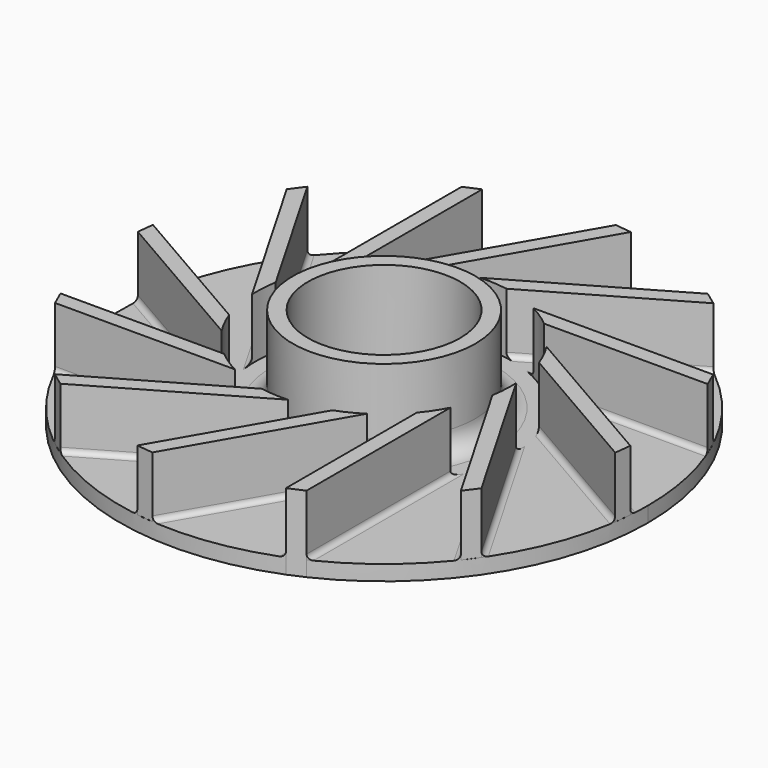
from build123d import *

# Parameters (mm, degrees)
F0_R          = 9
F0_R_2        = 7.5
F1_DEPTH      = 1.5
F2_DEPTH      = 7.5
F3_DEPTH      = 10
F4_COUNT      = 12
F6_T4_DEPTH   = 20.2062125085
F6_S5_R       = 26
F6_T6_DEPTH   = 12
F6_S7_R       = 12.5604672282
F6_T8_DEPTH   = 12
F6_T12_DEPTH  = 20.2062125085
F6_S13_R      = 26
F6_T14_DEPTH  = 12
F6_S15_R      = 12.5604672282
F6_T16_DEPTH  = 12
F6_T20_DEPTH  = 20.2062125085
F6_S21_R      = 26
F6_T22_DEPTH  = 12
F6_S23_R      = 12.5604672282
F6_T24_DEPTH  = 12
F6_T28_DEPTH  = 20.2062125085
F6_S29_R      = 26
F6_T30_DEPTH  = 12
F6_S31_R      = 12.5604672282
F6_T32_DEPTH  = 12
F6_T36_DEPTH  = 18.6035363085
F6_S37_R      = 12.5604672282
F6_T38_DEPTH  = 11
F6_S39_R      = 26
F6_T40_DEPTH  = 11
F6_T44_DEPTH  = 18.6035363085
F6_S45_R      = 12.5604672282
F6_T46_DEPTH  = 11
F6_S47_R      = 26
F6_T48_DEPTH  = 11
F6_T52_DEPTH  = 18.6035363085
F6_S53_R      = 12.5604672282
F6_T54_DEPTH  = 11
F6_S55_R      = 26
F6_T56_DEPTH  = 11
F6_T60_DEPTH  = 18.6035363085
F6_S61_R      = 12.5604672282
F6_T62_DEPTH  = 11
F6_S63_R      = 26
F6_T64_DEPTH  = 11
F6_T68_DEPTH  = 18.6035363085
F6_S69_R      = 12.5604672282
F6_T70_DEPTH  = 11
F6_S71_R      = 26
F6_T72_DEPTH  = 11
F6_T76_DEPTH  = 18.6035363085
F6_S77_R      = 12.5604672282
F6_T78_DEPTH  = 11
F6_S79_R      = 26
F6_T80_DEPTH  = 11
F6_T84_DEPTH  = 20.2062125085
F6_S85_R      = 26
F6_T86_DEPTH  = 12
F6_S87_R      = 12.5604672282
F6_T88_DEPTH  = 12
F6_T92_DEPTH  = 20.2062125085
F6_S93_R      = 26
F6_T94_DEPTH  = 12
F6_S95_R      = 12.5604672282
F6_T96_DEPTH  = 12
F6_T100_DEPTH = 20.2062125085
F6_S101_R     = 26
F6_T102_DEPTH = 12
F6_S103_R     = 12.5604672282
F6_T104_DEPTH = 12
F6_T108_DEPTH = 20.2062125085
F6_S109_R     = 26
F6_T110_DEPTH = 12
F6_S111_R     = 12.5604672282
F6_T112_DEPTH = 12
F6_T116_DEPTH = 20.2062125085
F6_S117_R     = 26
F6_T118_DEPTH = 12
F6_S119_R     = 12.5604672282
F6_T120_DEPTH = 12
F6_T124_DEPTH = 18.6035363085
F6_S125_R     = 12.5604672282
F6_T126_DEPTH = 11
F6_S127_R     = 26
F6_T128_DEPTH = 11
F6_T132_DEPTH = 18.6035363085
F6_S133_R     = 12.5604672282
F6_T134_DEPTH = 11
F6_S135_R     = 26
F6_T136_DEPTH = 11
F6_T140_DEPTH = 18.6035363085
F6_S141_R     = 12.5604672282
F6_T142_DEPTH = 11
F6_S143_R     = 26
F6_T144_DEPTH = 11
F6_T148_DEPTH = 18.6035363085
F6_S149_R     = 12.5604672282
F6_T150_DEPTH = 11
F6_S151_R     = 26
F6_T152_DEPTH = 11
F6_T156_DEPTH = 18.6035363085
F6_S157_R     = 12.5604672282
F6_T158_DEPTH = 11
F6_S159_R     = 26
F6_T160_DEPTH = 11
F6_T164_DEPTH = 18.6035363085
F6_S165_R     = 12.5604672282
F6_T166_DEPTH = 11
F6_S167_R     = 26
F6_T168_DEPTH = 11
F6_T172_DEPTH = 20.2062125085
F6_S173_R     = 26
F6_T174_DEPTH = 12
F6_S175_R     = 12.5604672282
F6_T176_DEPTH = 12
F6_T180_DEPTH = 20.2062125085
F6_S181_R     = 12.5604672282
F6_T182_DEPTH = 12
F6_S183_R     = 26
F6_T184_DEPTH = 12
F6_T188_DEPTH = 20.2062125085
F6_S189_R     = 26
F6_T190_DEPTH = 12
F6_S191_R     = 12.5604672282
F6_T192_DEPTH = 12
F7_R          = 2


# Not quite as in the source:
# - a fillet or chamfer that OpenCascade refuses, or shapes differently, is made with other operations: its cross-section is extruded or revolved along the edge and cut away or added


with BuildPart() as f1:
    # F0 (on Top) → F1 (new body)
    with BuildSketch(Plane.XY):
        with BuildLine():
            ThreePointArc((11.1509456635, -23.4873670472), (21.9764031094, -13.8938010053), (26, 0))
            ThreePointArc((26, 0), (-21.5281744146, 14.5786729977), (9.6509456635, -24.1424780791))
            Line((9.6509456635, -24.1424780791), (9.6509456635, -23.4873670472))
            Line((9.6509456635, -23.4873670472), (9.6509456635, -8.0389417706))
            ThreePointArc((9.6509456635, -8.0389417706), (10.462029989, -6.9506305829), (11.1509456635, -5.7811545388))
            Line((11.1509456635, -5.7811545388), (11.1509456635, -23.4873670472))
        make_face()
        Circle(F0_R, mode=Mode.SUBTRACT)
        Circle(F0_R)
        Circle(F0_R_2, mode=Mode.SUBTRACT)
    extrude(amount=F1_DEPTH)

    # F0 (on Top) → F3 (join)
    with BuildSketch(Plane.XY):
        Circle(F0_R)
        Circle(F0_R_2, mode=Mode.SUBTRACT)
    extrude(amount=F3_DEPTH)


with BuildPart() as f2:
    # F0 (on Top) → F2 (new body)
    with BuildSketch(Plane.XY):
        with BuildLine():
            Line((9.6509456635, -23.4873670472), (9.6509456635, -24.1424780791))
            Line((9.6509456635, -24.1424780791), (11.1509456635, -23.4873670472))
            Line((11.1509456635, -23.4873670472), (11.1509456635, -5.7811545388))
            ThreePointArc((11.1509456635, -5.7811545388), (10.462029989, -6.9506305829), (9.6509456635, -8.0389417706))
            Line((9.6509456635, -8.0389417706), (9.6509456635, -23.4873670472))
        make_face()
    extrude(amount=F2_DEPTH)


with BuildPart() as f4_1:
    # F4: instance of F2
    add(f2.part.rotate(Axis((0, 0, 0), (0, 0, 1)), 1 * 360 / F4_COUNT))


with BuildPart() as f4_2:
    # F4: instance of F2
    add(f2.part.rotate(Axis((0, 0, 0), (0, 0, 1)), 2 * 360 / F4_COUNT))


with BuildPart() as f4_3:
    # F4: instance of F2
    add(f2.part.rotate(Axis((0, 0, 0), (0, 0, 1)), 3 * 360 / F4_COUNT))


with BuildPart() as f4_4:
    # F4: instance of F2
    add(f2.part.rotate(Axis((0, 0, 0), (0, 0, 1)), 4 * 360 / F4_COUNT))


with BuildPart() as f4_5:
    # F4: instance of F2
    add(f2.part.rotate(Axis((0, 0, 0), (0, 0, 1)), 5 * 360 / F4_COUNT))


with BuildPart() as f4_6:
    # F4: instance of F2
    add(f2.part.rotate(Axis((0, 0, 0), (0, 0, 1)), 6 * 360 / F4_COUNT))


with BuildPart() as f4_7:
    # F4: instance of F2
    add(f2.part.rotate(Axis((0, 0, 0), (0, 0, 1)), 7 * 360 / F4_COUNT))


with BuildPart() as f4_8:
    # F4: instance of F2
    add(f2.part.rotate(Axis((0, 0, 0), (0, 0, 1)), 8 * 360 / F4_COUNT))


with BuildPart() as f4_9:
    # F4: instance of F2
    add(f2.part.rotate(Axis((0, 0, 0), (0, 0, 1)), 9 * 360 / F4_COUNT))


with BuildPart() as f4_10:
    # F4: instance of F2
    add(f2.part.rotate(Axis((0, 0, 0), (0, 0, 1)), 10 * 360 / F4_COUNT))


with BuildPart() as f4_11:
    # F4: instance of F2
    add(f2.part.rotate(Axis((0, 0, 0), (0, 0, 1)), 11 * 360 / F4_COUNT))


with BuildPart() as f1_1:
    add(f1.part)

    # F5: union F4_1, F4_2, F2, F4_3, F4_4, F4_5, F4_6, F4_7, F4_8, F4_9, F4_10, F4_11
    add(f4_1.part)
    add(f4_2.part)
    add(f2.part)
    add(f4_3.part)
    add(f4_4.part)
    add(f4_5.part)
    add(f4_6.part)
    add(f4_7.part)
    add(f4_8.part)
    add(f4_9.part)
    add(f4_10.part)
    add(f4_11.part)

    # F6: fillet of radius 0.5 on 24 edges, made by hand


with BuildPart() as f6_tool2:
    # F6_s3 → F6_t4 (new body)
    with BuildSketch(Plane(origin=(-2.2655772694, 3.924094939, 0), x_dir=(0, 0, 1), z_dir=(-0.5, 0.8660254038, 0))):
        with BuildLine():
            ThreePointArc((1.5, -11.6509456635), (1.6464466094, -11.2973922729), (2, -11.1509456635))
            Line((2, -11.1509456635), (1.5, -11.1509456635))
            Line((1.5, -11.1509456635), (1.5, -11.6509456635))
        make_face()
    extrude(amount=F6_T4_DEPTH)

    # F6_s5 → F6_t6 (intersect, symmetric)
    with BuildSketch(Plane.XY.offset(1.8)):
        Circle(F6_S5_R)
    extrude(amount=F6_T6_DEPTH, both=True, mode=Mode.INTERSECT)

    # F6_s7 → F6_t8 (cut, symmetric)
    with BuildSketch(Plane.XY.offset(1.8)):
        Circle(F6_S7_R)
    extrude(amount=F6_T8_DEPTH, both=True, mode=Mode.SUBTRACT)


with BuildPart() as f1_2:
    add(f1_1.part)

    # F6_t1: union F6_tool2
    add(f6_tool2.part)


with BuildPart() as f6_tool10:
    # F6_s11 → F6_t12 (new body)
    with BuildSketch(Plane(origin=(-3.924094939, 2.2655772694, 0), x_dir=(0, 0, 1), z_dir=(-0.8660254038, 0.5, 0))):
        with BuildLine():
            ThreePointArc((1.5, -11.6509456635), (1.6464466094, -11.2973922729), (2, -11.1509456635))
            Line((2, -11.1509456635), (1.5, -11.1509456635))
            Line((1.5, -11.1509456635), (1.5, -11.6509456635))
        make_face()
    extrude(amount=F6_T12_DEPTH)

    # F6_s13 → F6_t14 (intersect, symmetric)
    with BuildSketch(Plane.XY.offset(1.8)):
        Circle(F6_S13_R)
    extrude(amount=F6_T14_DEPTH, both=True, mode=Mode.INTERSECT)

    # F6_s15 → F6_t16 (cut, symmetric)
    with BuildSketch(Plane.XY.offset(1.8)):
        Circle(F6_S15_R)
    extrude(amount=F6_T16_DEPTH, both=True, mode=Mode.SUBTRACT)


with BuildPart() as f1_3:
    add(f1_2.part)

    # F6_t9: union F6_tool10
    add(f6_tool10.part)


with BuildPart() as f6_tool18:
    # F6_s19 → F6_t20 (new body)
    with BuildSketch(Plane.YZ.offset(-4.5311545388)):
        with BuildLine():
            ThreePointArc((-11.6509456635, 1.5), (-11.2973922729, 1.6464466094), (-11.1509456635, 2))
            Line((-11.1509456635, 2), (-11.1509456635, 1.5))
            Line((-11.1509456635, 1.5), (-11.6509456635, 1.5))
        make_face()
    extrude(amount=-F6_T20_DEPTH)

    # F6_s21 → F6_t22 (intersect, symmetric)
    with BuildSketch(Plane.XY.offset(1.8)):
        Circle(F6_S21_R)
    extrude(amount=F6_T22_DEPTH, both=True, mode=Mode.INTERSECT)

    # F6_s23 → F6_t24 (cut, symmetric)
    with BuildSketch(Plane.XY.offset(1.8)):
        Circle(F6_S23_R)
    extrude(amount=F6_T24_DEPTH, both=True, mode=Mode.SUBTRACT)


with BuildPart() as f1_4:
    add(f1_3.part)

    # F6_t17: union F6_tool18
    add(f6_tool18.part)


with BuildPart() as f6_tool26:
    # F6_s27 → F6_t28 (new body)
    with BuildSketch(Plane(origin=(-3.924094939, -2.2655772694, 0), x_dir=(0, 0, 1), z_dir=(-0.8660254038, -0.5, 0))):
        with BuildLine():
            ThreePointArc((1.5, -11.6509456635), (1.6464466094, -11.2973922729), (2, -11.1509456635))
            Line((2, -11.1509456635), (1.5, -11.1509456635))
            Line((1.5, -11.1509456635), (1.5, -11.6509456635))
        make_face()
    extrude(amount=F6_T28_DEPTH)

    # F6_s29 → F6_t30 (intersect, symmetric)
    with BuildSketch(Plane.XY.offset(1.8)):
        Circle(F6_S29_R)
    extrude(amount=F6_T30_DEPTH, both=True, mode=Mode.INTERSECT)

    # F6_s31 → F6_t32 (cut, symmetric)
    with BuildSketch(Plane.XY.offset(1.8)):
        Circle(F6_S31_R)
    extrude(amount=F6_T32_DEPTH, both=True, mode=Mode.SUBTRACT)


with BuildPart() as f1_5:
    add(f1_4.part)

    # F6_t25: union F6_tool26
    add(f6_tool26.part)


with BuildPart() as f6_tool34:
    # F6_s35 → F6_t36 (new body)
    with BuildSketch(Plane(origin=(-21.9905310816, 12.6962390396, 0), x_dir=(0, 0, 1), z_dir=(0.8660254038, -0.5, 0))):
        with BuildLine():
            ThreePointArc((1.5, 9.1509456635), (1.6464466094, 9.504499054), (2, 9.6509456635))
            Line((2, 9.6509456635), (1.5, 9.6509456635))
            Line((1.5, 9.6509456635), (1.5, 9.1509456635))
        make_face()
    extrude(amount=F6_T36_DEPTH)

    # F6_s37 → F6_t38 (cut, symmetric)
    with BuildSketch(Plane.XY.offset(1.8)):
        Circle(F6_S37_R)
    extrude(amount=F6_T38_DEPTH, both=True, mode=Mode.SUBTRACT)

    # F6_s39 → F6_t40 (intersect, symmetric)
    with BuildSketch(Plane.XY.offset(1.8)):
        Circle(F6_S39_R)
    extrude(amount=F6_T40_DEPTH, both=True, mode=Mode.INTERSECT)


with BuildPart() as f1_6:
    add(f1_5.part)

    # F6_t33: union F6_tool34
    add(f6_tool34.part)


with BuildPart() as f6_tool42:
    # F6_s43 → F6_t44 (new body)
    with BuildSketch(Plane.YZ.offset(-25.3924780791)):
        with BuildLine():
            ThreePointArc((-9.1509456635, 1.5), (-9.504499054, 1.6464466094), (-9.6509456635, 2))
            Line((-9.6509456635, 2), (-9.6509456635, 1.5))
            Line((-9.6509456635, 1.5), (-9.1509456635, 1.5))
        make_face()
    extrude(amount=F6_T44_DEPTH)

    # F6_s45 → F6_t46 (cut, symmetric)
    with BuildSketch(Plane.XY.offset(1.8)):
        Circle(F6_S45_R)
    extrude(amount=F6_T46_DEPTH, both=True, mode=Mode.SUBTRACT)

    # F6_s47 → F6_t48 (intersect, symmetric)
    with BuildSketch(Plane.XY.offset(1.8)):
        Circle(F6_S47_R)
    extrude(amount=F6_T48_DEPTH, both=True, mode=Mode.INTERSECT)


with BuildPart() as f1_7:
    add(f1_6.part)

    # F6_t41: union F6_tool42
    add(f6_tool42.part)


with BuildPart() as f6_tool50:
    # F6_s51 → F6_t52 (new body)
    with BuildSketch(Plane(origin=(-21.9905310816, -12.6962390396, 0), x_dir=(0, 0, 1), z_dir=(0.8660254038, 0.5, 0))):
        with BuildLine():
            ThreePointArc((1.5, 9.1509456635), (1.6464466094, 9.504499054), (2, 9.6509456635))
            Line((2, 9.6509456635), (1.5, 9.6509456635))
            Line((1.5, 9.6509456635), (1.5, 9.1509456635))
        make_face()
    extrude(amount=F6_T52_DEPTH)

    # F6_s53 → F6_t54 (cut, symmetric)
    with BuildSketch(Plane.XY.offset(1.8)):
        Circle(F6_S53_R)
    extrude(amount=F6_T54_DEPTH, both=True, mode=Mode.SUBTRACT)

    # F6_s55 → F6_t56 (intersect, symmetric)
    with BuildSketch(Plane.XY.offset(1.8)):
        Circle(F6_S55_R)
    extrude(amount=F6_T56_DEPTH, both=True, mode=Mode.INTERSECT)


with BuildPart() as f1_8:
    add(f1_7.part)

    # F6_t49: union F6_tool50
    add(f6_tool50.part)


with BuildPart() as f6_tool58:
    # F6_s59 → F6_t60 (new body)
    with BuildSketch(Plane(origin=(-12.6962390396, -21.9905310816, 0), x_dir=(0, 0, 1), z_dir=(0.5, 0.8660254038, 0))):
        with BuildLine():
            ThreePointArc((1.5, 9.1509456635), (1.6464466094, 9.504499054), (2, 9.6509456635))
            Line((2, 9.6509456635), (1.5, 9.6509456635))
            Line((1.5, 9.6509456635), (1.5, 9.1509456635))
        make_face()
    extrude(amount=F6_T60_DEPTH)

    # F6_s61 → F6_t62 (cut, symmetric)
    with BuildSketch(Plane.XY.offset(1.8)):
        Circle(F6_S61_R)
    extrude(amount=F6_T62_DEPTH, both=True, mode=Mode.SUBTRACT)

    # F6_s63 → F6_t64 (intersect, symmetric)
    with BuildSketch(Plane.XY.offset(1.8)):
        Circle(F6_S63_R)
    extrude(amount=F6_T64_DEPTH, both=True, mode=Mode.INTERSECT)


with BuildPart() as f1_9:
    add(f1_8.part)

    # F6_t57: union F6_tool58
    add(f6_tool58.part)


with BuildPart() as f6_tool66:
    # F6_s67 → F6_t68 (new body)
    with BuildSketch(Plane.XZ.offset(25.3924780791)):
        with BuildLine():
            ThreePointArc((9.1509456635, 1.5), (9.504499054, 1.6464466094), (9.6509456635, 2))
            Line((9.6509456635, 2), (9.6509456635, 1.5))
            Line((9.6509456635, 1.5), (9.1509456635, 1.5))
        make_face()
    extrude(amount=-F6_T68_DEPTH)

    # F6_s69 → F6_t70 (cut, symmetric)
    with BuildSketch(Plane.XY.offset(1.8)):
        Circle(F6_S69_R)
    extrude(amount=F6_T70_DEPTH, both=True, mode=Mode.SUBTRACT)

    # F6_s71 → F6_t72 (intersect, symmetric)
    with BuildSketch(Plane.XY.offset(1.8)):
        Circle(F6_S71_R)
    extrude(amount=F6_T72_DEPTH, both=True, mode=Mode.INTERSECT)


with BuildPart() as f1_10:
    add(f1_9.part)

    # F6_t65: union F6_tool66
    add(f6_tool66.part)


with BuildPart() as f6_tool74:
    # F6_s75 → F6_t76 (new body)
    with BuildSketch(Plane(origin=(12.6962390396, -21.9905310816, 0), x_dir=(0, 0, 1), z_dir=(-0.5, 0.8660254038, 0))):
        with BuildLine():
            ThreePointArc((1.5, 9.1509456635), (1.6464466094, 9.504499054), (2, 9.6509456635))
            Line((2, 9.6509456635), (1.5, 9.6509456635))
            Line((1.5, 9.6509456635), (1.5, 9.1509456635))
        make_face()
    extrude(amount=F6_T76_DEPTH)

    # F6_s77 → F6_t78 (cut, symmetric)
    with BuildSketch(Plane.XY.offset(1.8)):
        Circle(F6_S77_R)
    extrude(amount=F6_T78_DEPTH, both=True, mode=Mode.SUBTRACT)

    # F6_s79 → F6_t80 (intersect, symmetric)
    with BuildSketch(Plane.XY.offset(1.8)):
        Circle(F6_S79_R)
    extrude(amount=F6_T80_DEPTH, both=True, mode=Mode.INTERSECT)


with BuildPart() as f1_11:
    add(f1_10.part)

    # F6_t73: union F6_tool74
    add(f6_tool74.part)


with BuildPart() as f6_tool82:
    # F6_s83 → F6_t84 (new body)
    with BuildSketch(Plane(origin=(3.924094939, -2.2655772694, 0), x_dir=(0, 0, 1), z_dir=(0.8660254038, -0.5, 0))):
        with BuildLine():
            ThreePointArc((1.5, -11.6509456635), (1.6464466094, -11.2973922729), (2, -11.1509456635))
            Line((2, -11.1509456635), (1.5, -11.1509456635))
            Line((1.5, -11.1509456635), (1.5, -11.6509456635))
        make_face()
    extrude(amount=F6_T84_DEPTH)

    # F6_s85 → F6_t86 (intersect, symmetric)
    with BuildSketch(Plane.XY.offset(1.8)):
        Circle(F6_S85_R)
    extrude(amount=F6_T86_DEPTH, both=True, mode=Mode.INTERSECT)

    # F6_s87 → F6_t88 (cut, symmetric)
    with BuildSketch(Plane.XY.offset(1.8)):
        Circle(F6_S87_R)
    extrude(amount=F6_T88_DEPTH, both=True, mode=Mode.SUBTRACT)


with BuildPart() as f1_12:
    add(f1_11.part)

    # F6_t81: union F6_tool82
    add(f6_tool82.part)


with BuildPart() as f6_tool90:
    # F6_s91 → F6_t92 (new body)
    with BuildSketch(Plane.YZ.offset(4.5311545388)):
        with BuildLine():
            ThreePointArc((11.6509456635, 1.5), (11.2973922729, 1.6464466094), (11.1509456635, 2))
            Line((11.1509456635, 2), (11.1509456635, 1.5))
            Line((11.1509456635, 1.5), (11.6509456635, 1.5))
        make_face()
    extrude(amount=F6_T92_DEPTH)

    # F6_s93 → F6_t94 (intersect, symmetric)
    with BuildSketch(Plane.XY.offset(1.8)):
        Circle(F6_S93_R)
    extrude(amount=F6_T94_DEPTH, both=True, mode=Mode.INTERSECT)

    # F6_s95 → F6_t96 (cut, symmetric)
    with BuildSketch(Plane.XY.offset(1.8)):
        Circle(F6_S95_R)
    extrude(amount=F6_T96_DEPTH, both=True, mode=Mode.SUBTRACT)


with BuildPart() as f1_13:
    add(f1_12.part)

    # F6_t89: union F6_tool90
    add(f6_tool90.part)


with BuildPart() as f6_tool98:
    # F6_s99 → F6_t100 (new body)
    with BuildSketch(Plane(origin=(3.924094939, 2.2655772694, 0), x_dir=(0, 0, 1), z_dir=(0.8660254038, 0.5, 0))):
        with BuildLine():
            ThreePointArc((1.5, -11.6509456635), (1.6464466094, -11.2973922729), (2, -11.1509456635))
            Line((2, -11.1509456635), (1.5, -11.1509456635))
            Line((1.5, -11.1509456635), (1.5, -11.6509456635))
        make_face()
    extrude(amount=F6_T100_DEPTH)

    # F6_s101 → F6_t102 (intersect, symmetric)
    with BuildSketch(Plane.XY.offset(1.8)):
        Circle(F6_S101_R)
    extrude(amount=F6_T102_DEPTH, both=True, mode=Mode.INTERSECT)

    # F6_s103 → F6_t104 (cut, symmetric)
    with BuildSketch(Plane.XY.offset(1.8)):
        Circle(F6_S103_R)
    extrude(amount=F6_T104_DEPTH, both=True, mode=Mode.SUBTRACT)


with BuildPart() as f1_14:
    add(f1_13.part)

    # F6_t97: union F6_tool98
    add(f6_tool98.part)


with BuildPart() as f6_tool106:
    # F6_s107 → F6_t108 (new body)
    with BuildSketch(Plane(origin=(2.2655772694, 3.924094939, 0), x_dir=(0, 0, 1), z_dir=(0.5, 0.8660254038, 0))):
        with BuildLine():
            ThreePointArc((1.5, -11.6509456635), (1.6464466094, -11.2973922729), (2, -11.1509456635))
            Line((2, -11.1509456635), (1.5, -11.1509456635))
            Line((1.5, -11.1509456635), (1.5, -11.6509456635))
        make_face()
    extrude(amount=F6_T108_DEPTH)

    # F6_s109 → F6_t110 (intersect, symmetric)
    with BuildSketch(Plane.XY.offset(1.8)):
        Circle(F6_S109_R)
    extrude(amount=F6_T110_DEPTH, both=True, mode=Mode.INTERSECT)

    # F6_s111 → F6_t112 (cut, symmetric)
    with BuildSketch(Plane.XY.offset(1.8)):
        Circle(F6_S111_R)
    extrude(amount=F6_T112_DEPTH, both=True, mode=Mode.SUBTRACT)


with BuildPart() as f1_15:
    add(f1_14.part)

    # F6_t105: union F6_tool106
    add(f6_tool106.part)


with BuildPart() as f6_tool114:
    # F6_s115 → F6_t116 (new body)
    with BuildSketch(Plane.XZ.offset(-4.5311545388)):
        with BuildLine():
            ThreePointArc((-11.6509456635, 1.5), (-11.2973922729, 1.6464466094), (-11.1509456635, 2))
            Line((-11.1509456635, 2), (-11.1509456635, 1.5))
            Line((-11.1509456635, 1.5), (-11.6509456635, 1.5))
        make_face()
    extrude(amount=-F6_T116_DEPTH)

    # F6_s117 → F6_t118 (intersect, symmetric)
    with BuildSketch(Plane.XY.offset(1.8)):
        Circle(F6_S117_R)
    extrude(amount=F6_T118_DEPTH, both=True, mode=Mode.INTERSECT)

    # F6_s119 → F6_t120 (cut, symmetric)
    with BuildSketch(Plane.XY.offset(1.8)):
        Circle(F6_S119_R)
    extrude(amount=F6_T120_DEPTH, both=True, mode=Mode.SUBTRACT)


with BuildPart() as f1_16:
    add(f1_15.part)

    # F6_t113: union F6_tool114
    add(f6_tool114.part)


with BuildPart() as f6_tool122:
    # F6_s123 → F6_t124 (new body)
    with BuildSketch(Plane.XZ.offset(-25.3924780791)):
        with BuildLine():
            ThreePointArc((-9.1509456635, 1.5), (-9.504499054, 1.6464466094), (-9.6509456635, 2))
            Line((-9.6509456635, 2), (-9.6509456635, 1.5))
            Line((-9.6509456635, 1.5), (-9.1509456635, 1.5))
        make_face()
    extrude(amount=F6_T124_DEPTH)

    # F6_s125 → F6_t126 (cut, symmetric)
    with BuildSketch(Plane.XY.offset(1.8)):
        Circle(F6_S125_R)
    extrude(amount=F6_T126_DEPTH, both=True, mode=Mode.SUBTRACT)

    # F6_s127 → F6_t128 (intersect, symmetric)
    with BuildSketch(Plane.XY.offset(1.8)):
        Circle(F6_S127_R)
    extrude(amount=F6_T128_DEPTH, both=True, mode=Mode.INTERSECT)


with BuildPart() as f1_17:
    add(f1_16.part)

    # F6_t121: union F6_tool122
    add(f6_tool122.part)


with BuildPart() as f6_tool130:
    # F6_s131 → F6_t132 (new body)
    with BuildSketch(Plane(origin=(-12.6962390396, 21.9905310816, 0), x_dir=(0, 0, 1), z_dir=(0.5, -0.8660254038, 0))):
        with BuildLine():
            ThreePointArc((1.5, 9.1509456635), (1.6464466094, 9.504499054), (2, 9.6509456635))
            Line((2, 9.6509456635), (1.5, 9.6509456635))
            Line((1.5, 9.6509456635), (1.5, 9.1509456635))
        make_face()
    extrude(amount=F6_T132_DEPTH)

    # F6_s133 → F6_t134 (cut, symmetric)
    with BuildSketch(Plane.XY.offset(1.8)):
        Circle(F6_S133_R)
    extrude(amount=F6_T134_DEPTH, both=True, mode=Mode.SUBTRACT)

    # F6_s135 → F6_t136 (intersect, symmetric)
    with BuildSketch(Plane.XY.offset(1.8)):
        Circle(F6_S135_R)
    extrude(amount=F6_T136_DEPTH, both=True, mode=Mode.INTERSECT)


with BuildPart() as f1_18:
    add(f1_17.part)

    # F6_t129: union F6_tool130
    add(f6_tool130.part)


with BuildPart() as f6_tool138:
    # F6_s139 → F6_t140 (new body)
    with BuildSketch(Plane(origin=(12.6962390396, 21.9905310816, 0), x_dir=(0, 0, 1), z_dir=(-0.5, -0.8660254038, 0))):
        with BuildLine():
            ThreePointArc((1.5, 9.1509456635), (1.6464466094, 9.504499054), (2, 9.6509456635))
            Line((2, 9.6509456635), (1.5, 9.6509456635))
            Line((1.5, 9.6509456635), (1.5, 9.1509456635))
        make_face()
    extrude(amount=F6_T140_DEPTH)

    # F6_s141 → F6_t142 (cut, symmetric)
    with BuildSketch(Plane.XY.offset(1.8)):
        Circle(F6_S141_R)
    extrude(amount=F6_T142_DEPTH, both=True, mode=Mode.SUBTRACT)

    # F6_s143 → F6_t144 (intersect, symmetric)
    with BuildSketch(Plane.XY.offset(1.8)):
        Circle(F6_S143_R)
    extrude(amount=F6_T144_DEPTH, both=True, mode=Mode.INTERSECT)


with BuildPart() as f1_19:
    add(f1_18.part)

    # F6_t137: union F6_tool138
    add(f6_tool138.part)


with BuildPart() as f6_tool146:
    # F6_s147 → F6_t148 (new body)
    with BuildSketch(Plane(origin=(21.9905310816, 12.6962390396, 0), x_dir=(0, 0, 1), z_dir=(-0.8660254038, -0.5, 0))):
        with BuildLine():
            ThreePointArc((1.5, 9.1509456635), (1.6464466094, 9.504499054), (2, 9.6509456635))
            Line((2, 9.6509456635), (1.5, 9.6509456635))
            Line((1.5, 9.6509456635), (1.5, 9.1509456635))
        make_face()
    extrude(amount=F6_T148_DEPTH)

    # F6_s149 → F6_t150 (cut, symmetric)
    with BuildSketch(Plane.XY.offset(1.8)):
        Circle(F6_S149_R)
    extrude(amount=F6_T150_DEPTH, both=True, mode=Mode.SUBTRACT)

    # F6_s151 → F6_t152 (intersect, symmetric)
    with BuildSketch(Plane.XY.offset(1.8)):
        Circle(F6_S151_R)
    extrude(amount=F6_T152_DEPTH, both=True, mode=Mode.INTERSECT)


with BuildPart() as f1_20:
    add(f1_19.part)

    # F6_t145: union F6_tool146
    add(f6_tool146.part)


with BuildPart() as f6_tool154:
    # F6_s155 → F6_t156 (new body)
    with BuildSketch(Plane.YZ.offset(25.3924780791)):
        with BuildLine():
            ThreePointArc((9.1509456635, 1.5), (9.504499054, 1.6464466094), (9.6509456635, 2))
            Line((9.6509456635, 2), (9.6509456635, 1.5))
            Line((9.6509456635, 1.5), (9.1509456635, 1.5))
        make_face()
    extrude(amount=-F6_T156_DEPTH)

    # F6_s157 → F6_t158 (cut, symmetric)
    with BuildSketch(Plane.XY.offset(1.8)):
        Circle(F6_S157_R)
    extrude(amount=F6_T158_DEPTH, both=True, mode=Mode.SUBTRACT)

    # F6_s159 → F6_t160 (intersect, symmetric)
    with BuildSketch(Plane.XY.offset(1.8)):
        Circle(F6_S159_R)
    extrude(amount=F6_T160_DEPTH, both=True, mode=Mode.INTERSECT)


with BuildPart() as f1_21:
    add(f1_20.part)

    # F6_t153: union F6_tool154
    add(f6_tool154.part)


with BuildPart() as f6_tool162:
    # F6_s163 → F6_t164 (new body)
    with BuildSketch(Plane(origin=(21.9905310816, -12.6962390396, 0), x_dir=(0, 0, 1), z_dir=(-0.8660254038, 0.5, 0))):
        with BuildLine():
            ThreePointArc((1.5, 9.1509456635), (1.6464466094, 9.504499054), (2, 9.6509456635))
            Line((2, 9.6509456635), (1.5, 9.6509456635))
            Line((1.5, 9.6509456635), (1.5, 9.1509456635))
        make_face()
    extrude(amount=F6_T164_DEPTH)

    # F6_s165 → F6_t166 (cut, symmetric)
    with BuildSketch(Plane.XY.offset(1.8)):
        Circle(F6_S165_R)
    extrude(amount=F6_T166_DEPTH, both=True, mode=Mode.SUBTRACT)

    # F6_s167 → F6_t168 (intersect, symmetric)
    with BuildSketch(Plane.XY.offset(1.8)):
        Circle(F6_S167_R)
    extrude(amount=F6_T168_DEPTH, both=True, mode=Mode.INTERSECT)


with BuildPart() as f1_22:
    add(f1_21.part)

    # F6_t161: union F6_tool162
    add(f6_tool162.part)


with BuildPart() as f6_tool170:
    # F6_s171 → F6_t172 (new body)
    with BuildSketch(Plane(origin=(2.2655772694, -3.924094939, 0), x_dir=(0, 0, 1), z_dir=(0.5, -0.8660254038, 0))):
        with BuildLine():
            ThreePointArc((1.5, -11.6509456635), (1.6464466094, -11.2973922729), (2, -11.1509456635))
            Line((2, -11.1509456635), (1.5, -11.1509456635))
            Line((1.5, -11.1509456635), (1.5, -11.6509456635))
        make_face()
    extrude(amount=F6_T172_DEPTH)

    # F6_s173 → F6_t174 (intersect, symmetric)
    with BuildSketch(Plane.XY.offset(1.8)):
        Circle(F6_S173_R)
    extrude(amount=F6_T174_DEPTH, both=True, mode=Mode.INTERSECT)

    # F6_s175 → F6_t176 (cut, symmetric)
    with BuildSketch(Plane.XY.offset(1.8)):
        Circle(F6_S175_R)
    extrude(amount=F6_T176_DEPTH, both=True, mode=Mode.SUBTRACT)


with BuildPart() as f1_23:
    add(f1_22.part)

    # F6_t169: union F6_tool170
    add(f6_tool170.part)


with BuildPart() as f6_tool178:
    # F6_s179 → F6_t180 (new body)
    with BuildSketch(Plane.XZ.offset(4.5311545388)):
        with BuildLine():
            ThreePointArc((11.6509456635, 1.5), (11.2973922729, 1.6464466094), (11.1509456635, 2))
            Line((11.1509456635, 2), (11.1509456635, 1.5))
            Line((11.1509456635, 1.5), (11.6509456635, 1.5))
        make_face()
    extrude(amount=F6_T180_DEPTH)

    # F6_s181 → F6_t182 (cut, symmetric)
    with BuildSketch(Plane.XY.offset(1.8)):
        Circle(F6_S181_R)
    extrude(amount=F6_T182_DEPTH, both=True, mode=Mode.SUBTRACT)

    # F6_s183 → F6_t184 (intersect, symmetric)
    with BuildSketch(Plane.XY.offset(1.8)):
        Circle(F6_S183_R)
    extrude(amount=F6_T184_DEPTH, both=True, mode=Mode.INTERSECT)


with BuildPart() as f1_24:
    add(f1_23.part)

    # F6_t177: union F6_tool178
    add(f6_tool178.part)


with BuildPart() as f6_tool186:
    # F6_s187 → F6_t188 (new body)
    with BuildSketch(Plane(origin=(-2.2655772694, -3.924094939, 0), x_dir=(0, 0, 1), z_dir=(-0.5, -0.8660254038, 0))):
        with BuildLine():
            ThreePointArc((1.5, -11.6509456635), (1.6464466094, -11.2973922729), (2, -11.1509456635))
            Line((2, -11.1509456635), (1.5, -11.1509456635))
            Line((1.5, -11.1509456635), (1.5, -11.6509456635))
        make_face()
    extrude(amount=F6_T188_DEPTH)

    # F6_s189 → F6_t190 (intersect, symmetric)
    with BuildSketch(Plane.XY.offset(1.8)):
        Circle(F6_S189_R)
    extrude(amount=F6_T190_DEPTH, both=True, mode=Mode.INTERSECT)

    # F6_s191 → F6_t192 (cut, symmetric)
    with BuildSketch(Plane.XY.offset(1.8)):
        Circle(F6_S191_R)
    extrude(amount=F6_T192_DEPTH, both=True, mode=Mode.SUBTRACT)


with BuildPart() as f1_25:
    add(f1_24.part)

    # F6_t185: union F6_tool186
    add(f6_tool186.part)

    # F7
    f7_edges = [f1_25.edges().sort_by_distance(p)[0] for p in [
        (-9, 0, 1.5),
    ]]
    fillet(f7_edges, radius=F7_R)


solid = f1_25.part
